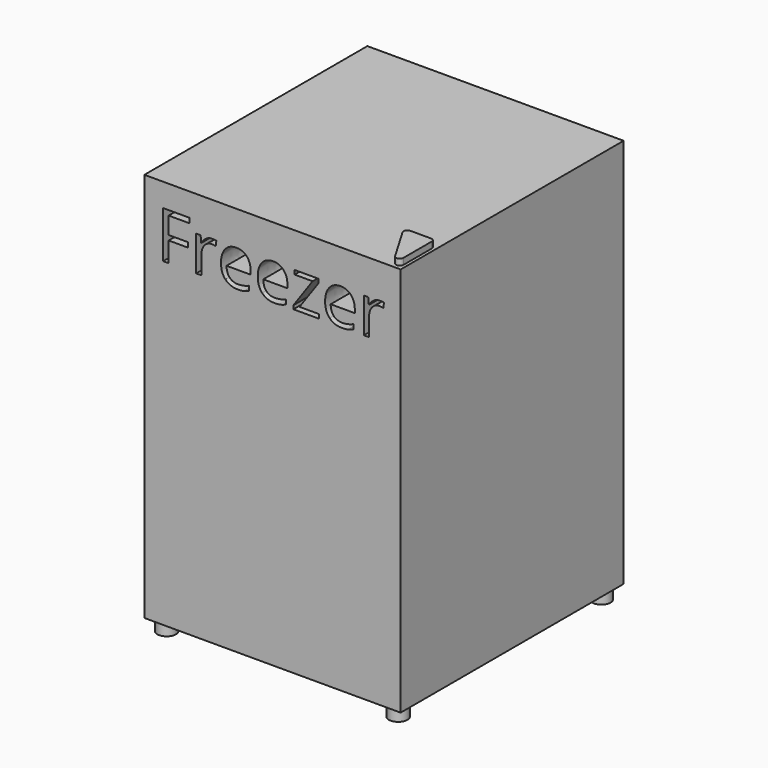
from build123d import *

# Parameters (mm, degrees)
F0_W        = 525.4625
F0_H        = 800.1
F1_DEPTH    = 571.5
F2_R        = 19.05
F3_DEPTH    = 25.4
F5_DEPTH    = 12.7
F6_T1_DEPTH = 82.6574729689
F6_T3_DEPTH = 31.75
F6_T5_DEPTH = 46.0073370405


# Not quite as in the source:
# - a fillet or chamfer that OpenCascade refuses, or shapes differently, is made with other operations: its cross-section is extruded or revolved along the edge and cut away or added


with BuildPart() as f1:
    # F0 (on Front) → F1 (new body)
    with BuildSketch(Plane.XZ):
        with Locations((262.73125, 474.3377777734)):
            Rectangle(F0_W, F0_H)
        with BuildLine():
            add(Edge.make_bspline(
                [(126.6487428161, 800.3234279035), (132.2934913793, 804.132059369), (139.0504022989, 804.132059369)],
                knots=[0, 0, 0, 1, 1, 1], degree=2))
            add(Edge.make_bspline(
                [(139.0504022989, 804.132059369), (143.8347988506, 804.132059369), (147.6329382184, 803.3346599437)],
                knots=[0, 0, 0, 1, 1, 1], degree=2))
            Line((147.6329382184, 803.3346599437), (146.1220761494, 793.2412619552))
            add(Edge.make_bspline(
                [(146.1220761494, 793.2412619552), (141.6734267241, 794.2275191391), (138.2530028736, 794.2275191391)],
                knots=[0, 0, 0, 1, 1, 1], degree=2))
            add(Edge.make_bspline(
                [(138.2530028736, 794.2275191391), (129.5235775862, 794.2275191391), (123.3332399425, 787.1453531909)],
                knots=[0, 0, 0, 1, 1, 1], degree=2))
            add(Edge.make_bspline(
                [(123.3332399425, 787.1453531909), (117.1429022989, 780.0631872426), (117.1429022989, 769.5081369552)],
                knots=[0, 0, 0, 1, 1, 1], degree=2))
            Line((117.1429022989, 769.5081369552), (117.1429022989, 730.9391858058))
            Line((117.1429022989, 730.9391858058), (106.2521048851, 730.9391858058))
            Line((106.2521048851, 730.9391858058), (106.2521048851, 802.8100550587))
            Line((106.2521048851, 802.8100550587), (115.2333405172, 802.8100550587))
            Line((115.2333405172, 802.8100550587), (116.4923922414, 789.5060751736))
            Line((116.4923922414, 789.5060751736), (117.0169971264, 789.5060751736))
            add(Edge.make_bspline(
                [(117.0169971264, 789.5060751736), (121.0039942529, 796.514796438), (126.6487428161, 800.3234279035)],
                knots=[0, 0, 0, 1, 1, 1], degree=2))
        make_face(mode=Mode.SUBTRACT)
        Polygon((49.7206824713, 771.9213194265), (49.7206824713, 730.9391858058), (38.5780747126, 730.9391858058), (38.5780747126, 826.8159745989), (92.0248204023, 826.8159745989), (92.0248204023, 816.911434369), (49.7206824713, 816.911434369), (49.7206824713, 781.8258596564), (89.4647485632, 781.8258596564), (89.4647485632, 771.9213194265), align=None, mode=Mode.SUBTRACT)
        with BuildLine():
            add(Edge.make_bspline(
                [(203.8705818966, 730.7083596564), (198.729454023, 729.6171814955), (191.4479382184, 729.6171814955)],
                knots=[0, 0, 0, 1, 1, 1], degree=2))
            add(Edge.make_bspline(
                [(191.4479382184, 729.6171814955), (175.520933908, 729.6171814955), (166.2983800287, 739.3328639667)],
                knots=[0, 0, 0, 1, 1, 1], degree=2))
            add(Edge.make_bspline(
                [(166.2983800287, 739.3328639667), (157.0758261494, 749.048546438), (157.0758261494, 766.2765708633)],
                knots=[0, 0, 0, 1, 1, 1], degree=2))
            add(Edge.make_bspline(
                [(157.0758261494, 766.2765708633), (157.0758261494, 783.6724688518), (165.6373778736, 793.9022641104)],
                knots=[0, 0, 0, 1, 1, 1], degree=2))
            add(Edge.make_bspline(
                [(165.6373778736, 793.9022641104), (174.1989295977, 804.132059369), (188.6360560345, 804.132059369)],
                knots=[0, 0, 0, 1, 1, 1], degree=2))
            add(Edge.make_bspline(
                [(188.6360560345, 804.132059369), (202.1288936782, 804.132059369), (209.997966954, 795.2452526162)],
                knots=[0, 0, 0, 1, 1, 1], degree=2))
            add(Edge.make_bspline(
                [(209.997966954, 795.2452526162), (217.8670402299, 786.3584458633), (217.8670402299, 771.7954142541)],
                knots=[0, 0, 0, 1, 1, 1], degree=2))
            Line((217.8670402299, 771.7954142541), (217.8670402299, 764.9125981621))
            Line((217.8670402299, 764.9125981621), (168.3653232759, 764.9125981621))
            add(Edge.make_bspline(
                [(168.3653232759, 764.9125981621), (168.7010704023, 752.2591283346), (174.7655028736, 745.7015672713)],
                knots=[0, 0, 0, 1, 1, 1], degree=2))
            add(Edge.make_bspline(
                [(174.7655028736, 745.7015672713), (180.8299353448, 739.1440062081), (191.846637931, 739.1440062081)],
                knots=[0, 0, 0, 1, 1, 1], degree=2))
            add(Edge.make_bspline(
                [(191.846637931, 739.1440062081), (203.4508979885, 739.1440062081), (214.7823635057, 743.991355346)],
                knots=[0, 0, 0, 1, 1, 1], degree=2))
            Line((214.7823635057, 743.991355346), (214.7823635057, 734.2756728748))
            add(Edge.make_bspline(
                [(214.7823635057, 734.2756728748), (209.0117097701, 731.7995378173), (203.8705818966, 730.7083596564)],
                knots=[0, 0, 0, 1, 1, 1], degree=2))
        make_face(mode=Mode.SUBTRACT)
        with BuildLine():
            add(Edge.make_bspline(
                [(279.2248275862, 730.7083596564), (274.0836997126, 729.6171814955), (266.802183908, 729.6171814955)],
                knots=[0, 0, 0, 1, 1, 1], degree=2))
            add(Edge.make_bspline(
                [(266.802183908, 729.6171814955), (250.8751795977, 729.6171814955), (241.6526257184, 739.3328639667)],
                knots=[0, 0, 0, 1, 1, 1], degree=2))
            add(Edge.make_bspline(
                [(241.6526257184, 739.3328639667), (232.4300718391, 749.048546438), (232.4300718391, 766.2765708633)],
                knots=[0, 0, 0, 1, 1, 1], degree=2))
            add(Edge.make_bspline(
                [(232.4300718391, 766.2765708633), (232.4300718391, 783.6724688518), (240.9916235632, 793.9022641104)],
                knots=[0, 0, 0, 1, 1, 1], degree=2))
            add(Edge.make_bspline(
                [(240.9916235632, 793.9022641104), (249.5531752874, 804.132059369), (263.9903017241, 804.132059369)],
                knots=[0, 0, 0, 1, 1, 1], degree=2))
            add(Edge.make_bspline(
                [(263.9903017241, 804.132059369), (277.4831393678, 804.132059369), (285.3522126437, 795.2452526162)],
                knots=[0, 0, 0, 1, 1, 1], degree=2))
            add(Edge.make_bspline(
                [(285.3522126437, 795.2452526162), (293.2212859195, 786.3584458633), (293.2212859195, 771.7954142541)],
                knots=[0, 0, 0, 1, 1, 1], degree=2))
            Line((293.2212859195, 771.7954142541), (293.2212859195, 764.9125981621))
            Line((293.2212859195, 764.9125981621), (243.7195689655, 764.9125981621))
            add(Edge.make_bspline(
                [(243.7195689655, 764.9125981621), (244.055316092, 752.2591283346), (250.1197485632, 745.7015672713)],
                knots=[0, 0, 0, 1, 1, 1], degree=2))
            add(Edge.make_bspline(
                [(250.1197485632, 745.7015672713), (256.1841810345, 739.1440062081), (267.2008836207, 739.1440062081)],
                knots=[0, 0, 0, 1, 1, 1], degree=2))
            add(Edge.make_bspline(
                [(267.2008836207, 739.1440062081), (278.8051436782, 739.1440062081), (290.1366091954, 743.991355346)],
                knots=[0, 0, 0, 1, 1, 1], degree=2))
            Line((290.1366091954, 743.991355346), (290.1366091954, 734.2756728748))
            add(Edge.make_bspline(
                [(290.1366091954, 734.2756728748), (284.3659554598, 731.7995378173), (279.2248275862, 730.7083596564)],
                knots=[0, 0, 0, 1, 1, 1], degree=2))
        make_face(mode=Mode.SUBTRACT)
        Polygon((357.768670977, 739.3958165529), (357.768670977, 730.9391858058), (305.6229454023, 730.9391858058), (305.6229454023, 738.3466067828), (344.8424066092, 794.3534243116), (308.057112069, 794.3534243116), (308.057112069, 802.8100550587), (356.7824137931, 802.8100550587), (356.7824137931, 794.3534243116), (318.0875574713, 739.3958165529), align=None, mode=Mode.SUBTRACT)
        with BuildLine():
            add(Edge.make_bspline(
                [(417.4057543103, 730.7083596564), (412.2646264368, 729.6171814955), (404.9831106322, 729.6171814955)],
                knots=[0, 0, 0, 1, 1, 1], degree=2))
            add(Edge.make_bspline(
                [(404.9831106322, 729.6171814955), (389.0561063218, 729.6171814955), (379.8335524425, 739.3328639667)],
                knots=[0, 0, 0, 1, 1, 1], degree=2))
            add(Edge.make_bspline(
                [(379.8335524425, 739.3328639667), (370.6109985632, 749.048546438), (370.6109985632, 766.2765708633)],
                knots=[0, 0, 0, 1, 1, 1], degree=2))
            add(Edge.make_bspline(
                [(370.6109985632, 766.2765708633), (370.6109985632, 783.6724688518), (379.1725502874, 793.9022641104)],
                knots=[0, 0, 0, 1, 1, 1], degree=2))
            add(Edge.make_bspline(
                [(379.1725502874, 793.9022641104), (387.7341020115, 804.132059369), (402.1712284483, 804.132059369)],
                knots=[0, 0, 0, 1, 1, 1], degree=2))
            add(Edge.make_bspline(
                [(402.1712284483, 804.132059369), (415.664066092, 804.132059369), (423.5331393678, 795.2452526162)],
                knots=[0, 0, 0, 1, 1, 1], degree=2))
            add(Edge.make_bspline(
                [(423.5331393678, 795.2452526162), (431.4022126437, 786.3584458633), (431.4022126437, 771.7954142541)],
                knots=[0, 0, 0, 1, 1, 1], degree=2))
            Line((431.4022126437, 771.7954142541), (431.4022126437, 764.9125981621))
            Line((431.4022126437, 764.9125981621), (381.9004956897, 764.9125981621))
            add(Edge.make_bspline(
                [(381.9004956897, 764.9125981621), (382.2362428161, 752.2591283346), (388.3006752874, 745.7015672713)],
                knots=[0, 0, 0, 1, 1, 1], degree=2))
            add(Edge.make_bspline(
                [(388.3006752874, 745.7015672713), (394.3651077586, 739.1440062081), (405.3818103448, 739.1440062081)],
                knots=[0, 0, 0, 1, 1, 1], degree=2))
            add(Edge.make_bspline(
                [(405.3818103448, 739.1440062081), (416.9860704023, 739.1440062081), (428.3175359195, 743.991355346)],
                knots=[0, 0, 0, 1, 1, 1], degree=2))
            Line((428.3175359195, 743.991355346), (428.3175359195, 734.2756728748))
            add(Edge.make_bspline(
                [(428.3175359195, 734.2756728748), (422.5468821839, 731.7995378173), (417.4057543103, 730.7083596564)],
                knots=[0, 0, 0, 1, 1, 1], degree=2))
        make_face(mode=Mode.SUBTRACT)
        with BuildLine():
            add(Edge.make_bspline(
                [(470.3698635057, 800.3234279035), (476.014612069, 804.132059369), (482.7715229885, 804.132059369)],
                knots=[0, 0, 0, 1, 1, 1], degree=2))
            add(Edge.make_bspline(
                [(482.7715229885, 804.132059369), (487.5559195402, 804.132059369), (491.354058908, 803.3346599437)],
                knots=[0, 0, 0, 1, 1, 1], degree=2))
            Line((491.354058908, 803.3346599437), (489.8431968391, 793.2412619552))
            add(Edge.make_bspline(
                [(489.8431968391, 793.2412619552), (485.3945474138, 794.2275191391), (481.9741235632, 794.2275191391)],
                knots=[0, 0, 0, 1, 1, 1], degree=2))
            add(Edge.make_bspline(
                [(481.9741235632, 794.2275191391), (473.2446982759, 794.2275191391), (467.0543606322, 787.1453531909)],
                knots=[0, 0, 0, 1, 1, 1], degree=2))
            add(Edge.make_bspline(
                [(467.0543606322, 787.1453531909), (460.8640229885, 780.0631872426), (460.8640229885, 769.5081369552)],
                knots=[0, 0, 0, 1, 1, 1], degree=2))
            Line((460.8640229885, 769.5081369552), (460.8640229885, 730.9391858058))
            Line((460.8640229885, 730.9391858058), (449.9732255747, 730.9391858058))
            Line((449.9732255747, 730.9391858058), (449.9732255747, 802.8100550587))
            Line((449.9732255747, 802.8100550587), (458.9544612069, 802.8100550587))
            Line((458.9544612069, 802.8100550587), (460.213512931, 789.5060751736))
            Line((460.213512931, 789.5060751736), (460.7381178161, 789.5060751736))
            add(Edge.make_bspline(
                [(460.7381178161, 789.5060751736), (464.7251149425, 796.514796438), (470.3698635057, 800.3234279035)],
                knots=[0, 0, 0, 1, 1, 1], degree=2))
        make_face(mode=Mode.SUBTRACT)
    extrude(amount=F1_DEPTH)

    # F2 (on face) → F3 (join)
    with BuildSketch(Plane(origin=(0, 0, 74.2877777734), x_dir=(1, 0, 0), z_dir=(0, 0, -1))):
        with Locations((25.4, 25.4)):
            Circle(F2_R)
        with Locations((25.4, 546.1)):
            Circle(F2_R)
        with Locations((500.0625, 546.1)):
            Circle(F2_R)
        with Locations((500.0625, 25.4)):
            Circle(F2_R)
    extrude(amount=F3_DEPTH)

    # F4 (on face) → F5 (join)
    with BuildSketch(Plane.XY.offset(874.3877777734)):
        Polygon((519.1125, -476.25), (455.6125, -476.25), (519.1125, -584.2), align=None)
    extrude(amount=F5_DEPTH)

    # F6: fillet of radius 7.62 on 3 edges, made by hand

    # F6_s2 → F6_t1 (cut)
    with BuildSketch(Plane.XY.offset(874.3877777734)):
        with BuildLine():
            ThreePointArc((504.9245612805, -560.0805041768), (513.4945872805, -563.5692925345), (519.1125, -556.2170108124))
            Line((519.1125, -556.2170108124), (519.1125, -584.2))
            Line((519.1125, -584.2), (504.9245612805, -560.0805041768))
        make_face()
    extrude(amount=F6_T1_DEPTH, mode=Mode.SUBTRACT)

    # F6_s4 → F6_t3 (cut)
    with BuildSketch(Plane.XY.offset(874.3877777734)):
        with BuildLine():
            ThreePointArc((511.4925, -476.25), (516.8806536726, -478.4818463274), (519.1125, -483.87))
            Line((519.1125, -483.87), (519.1125, -476.25))
            Line((519.1125, -476.25), (511.4925, -476.25))
        make_face()
    extrude(amount=F6_T3_DEPTH, mode=Mode.SUBTRACT)

    # F6_s6 → F6_t5 (cut)
    with BuildSketch(Plane.XY.offset(874.3877777734)):
        with BuildLine():
            ThreePointArc((462.3674960967, -487.7334933644), (462.3208970608, -480.0868412297), (468.9354348162, -476.25))
            Line((468.9354348162, -476.25), (455.6125, -476.25))
            Line((455.6125, -476.25), (462.3674960967, -487.7334933644))
        make_face()
    extrude(amount=F6_T5_DEPTH, mode=Mode.SUBTRACT)


solid = f1.part
